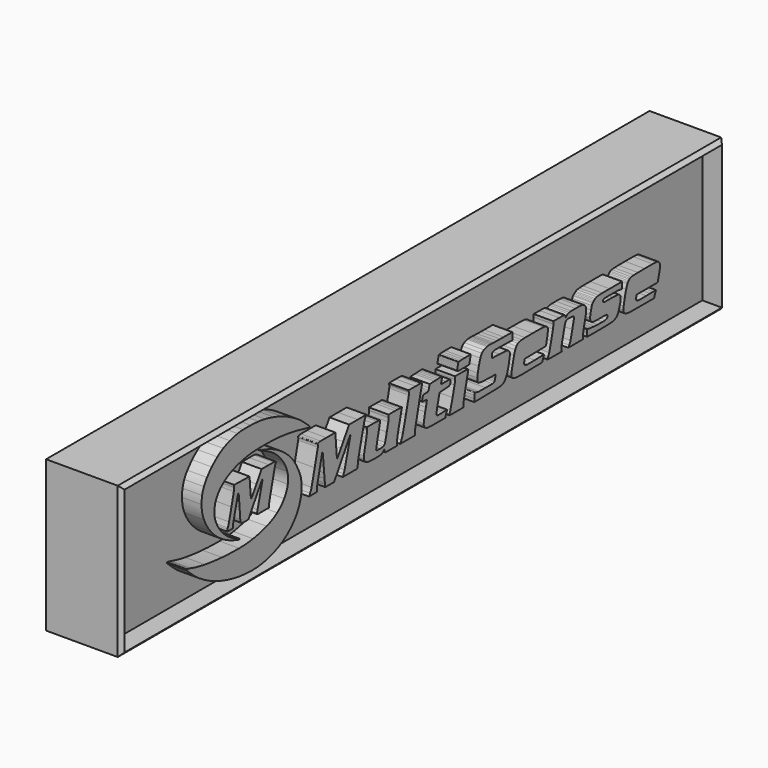
from build123d import *

# Parameters (mm, degrees)
F0_W     = 1000
F0_H     = 200
F1_DEPTH = 100
F2_SIZE  = 5
F3_W     = 990
F3_H     = 190
F4_DEPTH = 26


# Not quite as in the source:
# - ends of sketch curves that miss each other by under 0.0002 mm in the source are joined
# - a feature names something its author has since deleted; it is built from what else it names


with BuildPart() as f1:
    # F0 (on Right) → F1 (new body)
    with BuildSketch(Plane.YZ):
        Rectangle(F0_W, F0_H)
    extrude(amount=F1_DEPTH)

    # F2
    f2_edges = [f1.edges().sort_by_distance(p)[0] for p in [
        (100, 0, 100),
        (100, -500, 0),
        (100, 0, -100),
        (100, 500, 0),
    ]]
    chamfer(f2_edges, length=F2_SIZE)

    # F3 (on face) → F4 (cut)
    with BuildSketch(Plane.YZ.offset(100)):
        Rectangle(F3_W, F3_H)
        with BuildLine():
            ThreePointArc((-246.6238000578, 36.1891009246), (-255.0022324585, 41.7724397208), (-264.0417310007, 46.2063169983))
            ThreePointArc((-264.0417310007, 46.2063169983), (-266.1311900085, 47.0822687591), (-268.2084582005, 47.9867505481))
            ThreePointArc((-268.2084582005, 47.9867505481), (-268.3872731234, 48.2435637092), (-268.2422412968, 48.5208604908))
            ThreePointArc((-268.2422412968, 48.5208604908), (-267.7219027868, 48.7040052158), (-267.1717190083, 48.664106971))
            ThreePointArc((-267.1717190083, 48.664106971), (-264.7541220183, 47.9610524258), (-262.3439659438, 47.2328981825))
            ThreePointArc((-262.3439659438, 47.2328981825), (-255.75593138, 44.9664178565), (-249.3303629782, 42.2736120476))
            ThreePointArc((-249.3303629782, 42.2736120476), (-243.2724946687, 39.2332779494), (-237.4459938241, 35.7701452733))
            ThreePointArc((-237.4459938241, 35.7701452733), (-231.9833169046, 31.9676435498), (-226.8105147999, 27.7793292296))
            ThreePointArc((-226.8105147999, 27.7793292296), (-221.9912407206, 23.2545941628), (-217.5197788497, 18.3858511281))
            ThreePointArc((-217.5197788497, 18.3858511281), (-215.1211615749, 15.3479015259), (-212.9571917947, 12.1385811275))
            ThreePointArc((-212.9571917947, 12.1385811275), (-210.551378863, 8.0777492735), (-208.3170854587, 3.9200787657))
            ThreePointArc((-208.3170854587, 3.9200787657), (-206.3034941374, -0.2333235715), (-204.4645975596, -4.4669698195))
            ThreePointArc((-204.4645975596, -4.4669698195), (-203.2897357301, -7.7656038054), (-202.4281872957, -11.1595720605))
            ThreePointArc((-202.4281872957, -11.1595720605), (-201.4259177378, -22.427417277), (-202.9762712082, -33.6330089467))
            ThreePointArc((-202.9762712082, -33.6330089467), (-207.0222607184, -44.6408161639), (-213.2073987966, -54.6050481569))
            ThreePointArc((-213.2073987966, -54.6050481569), (-221.8366037995, -63.8856917917), (-232.0161676249, -71.4335396171))
            ThreePointArc((-232.0161676249, -71.4335396171), (-244.1370514451, -77.6181065611), (-257.0404061571, -81.9387693814))
            ThreePointArc((-257.0404061571, -81.9387693814), (-270.6114261246, -84.4639864171), (-284.3949819924, -85.2142472745))
            ThreePointArc((-284.3949819924, -85.2142472745), (-299.6324440177, -84.3227142054), (-314.7141769617, -81.9740098137))
            ThreePointArc((-314.7141769617, -81.9740098137), (-330.0151774272, -78.0817139303), (-344.8877120438, -72.782818107))
            ThreePointArc((-344.8877120438, -72.782818107), (-358.728779644, -66.2660528114), (-371.8313622416, -58.368856358))
            ThreePointArc((-371.8313622416, -58.368856358), (-374.9598139965, -56.1511961597), (-377.9827638038, -53.7917467602))
            ThreePointArc((-377.9827638038, -53.7917467602), (-381.6312348274, -50.7314998561), (-385.2042696474, -47.5835046094))
            ThreePointArc((-385.2042696474, -47.5835046094), (-388.7304292554, -44.3731215462), (-392.2297245717, -41.1334775412))
            ThreePointArc((-392.2297245717, -41.1334775412), (-392.4946359393, -40.5378059234), (-392.2503369729, -39.9333880271))
            ThreePointArc((-392.2503369729, -39.9333880271), (-392.0561404098, -39.8152470349), (-391.8293690277, -39.7996141612))
            ThreePointArc((-391.8293690277, -39.7996141612), (-390.9140495548, -39.9639754318), (-390.0013508704, -40.1423163625))
            ThreePointArc((-390.0013508704, -40.1423163625), (-388.9004354267, -40.3814829677), (-387.8062738459, -40.6498594061))
            ThreePointArc((-387.8062738459, -40.6498594061), (-386.5485933112, -40.9877691973), (-385.2969390093, -41.3473590314))
            ThreePointArc((-385.2969390093, -41.3473590314), (-373.7956362594, -44.3337818819), (-362.1164649515, -46.5236776815))
            ThreePointArc((-362.1164649515, -46.5236776815), (-347.8641152603, -48.4083534741), (-333.5490410005, -49.7350500068))
            ThreePointArc((-333.5490410005, -49.7350500068), (-319.2853989301, -50.496519542), (-305.0028930005, -50.6998549053))
            ThreePointArc((-305.0028930005, -50.6998549053), (-293.441650452, -50.2168691086), (-281.9462639341, -48.8933534329))
            ThreePointArc((-281.9462639341, -48.8933534329), (-270.522988434, -46.6581983207), (-259.3285238155, -43.4689815573))
            ThreePointArc((-259.3285238155, -43.4689815573), (-250.3750955195, -39.7652434038), (-242.0511392763, -34.8060796045))
            ThreePointArc((-242.0511392763, -34.8060796045), (-235.7079253752, -29.4741069957), (-230.4110620023, -23.1015459984))
            ThreePointArc((-230.4110620023, -23.1015459984), (-226.6480526025, -16.2091628127), (-224.3981197798, -8.6856670414))
            ThreePointArc((-224.3981197798, -8.6856670414), (-223.9008357191, -1.0084254056), (-225.2628372448, 6.5633829245))
            ThreePointArc((-225.2628372448, 6.5633829245), (-228.5350244194, 14.7357690405), (-233.0907067004, 22.2684222164))
            ThreePointArc((-233.0907067004, 22.2684222164), (-239.3489333395, 29.7229287703), (-246.6238000578, 36.1891009246))
        make_face(mode=Mode.SUBTRACT)
        with BuildLine():
            ThreePointArc((-174.7018401151, 14.0705920271), (-174.5288066312, 15.8520182991), (-174.8362170291, 17.6152309908))
            ThreePointArc((-174.8362170291, 17.6152309908), (-174.8622722087, 18.2073855305), (-174.5871220561, 18.7323790518))
            ThreePointArc((-174.5871220561, 18.7323790518), (-174.0368384738, 19.1539275213), (-173.3770499191, 19.3665164291))
            ThreePointArc((-173.3770499191, 19.3665164291), (-171.798102369, 19.5368741513), (-170.2113269933, 19.6019971351))
            ThreePointArc((-170.2113269933, 19.6019971351), (-165.3776001532, 19.6302348378), (-160.5438, 19.6396489998))
            Line((-160.5438, 19.6396489998), (-145.608858, 19.639649))
            Line((-145.608858, 19.639649), (-144.343966, 3.639649))
            ThreePointArc((-144.343966, 3.639649), (-144.0962884679, 0.5716718243), (-143.8384015545, -2.4954640475))
            ThreePointArc((-143.8384015545, -2.4954640475), (-143.6096761479, -5.0785607207), (-143.36664886, -7.6603510834))
            ThreePointArc((-143.36664886, -7.6603510834), (-143.1436912653, -9.9532312874), (-142.919313494, -12.2459729503))
            ThreePointArc((-142.919313494, -12.2459729503), (-142.8783010175, -12.327499768), (-142.793157, -12.360351))
            ThreePointArc((-142.793157, -12.360351), (-142.6920587596, -12.3343745217), (-142.6160043003, -12.2628808097))
            ThreePointArc((-142.6160043003, -12.2628808097), (-141.1591567944, -9.9628213076), (-139.7031838583, -7.6622080896))
            ThreePointArc((-139.7031838583, -7.6622080896), (-138.0793333583, -5.0838383234), (-136.4658248264, -2.4989841079))
            ThreePointArc((-136.4658248264, -2.4989841079), (-134.5669888164, 0.5648690609), (-132.6756031958, 3.6333271203))
            Line((-132.6756031958, 3.6333271203), (-122.843966, 19.627006))
            Line((-122.843966, 19.627006), (-108.570914, 19.633327))
            Line((-108.570914, 19.633327), (-94.297861, 19.639649))
            Line((-94.297861, 19.639649), (-95.759344, 17.389649))
            ThreePointArc((-95.759344, 17.389649), (-96.8435272527, 15.3828466119), (-97.5910089736, 13.2278569932))
            ThreePointArc((-97.5910089736, 13.2278569932), (-100.2300256588, 2.944764842), (-102.8292478626, -7.3484580344))
            ThreePointArc((-102.8292478626, -7.3484580344), (-105.3240499629, -17.4199326533), (-107.7666081157, -27.5042049723))
            ThreePointArc((-107.7666081157, -27.5042049723), (-108.3156162068, -30.5257876099), (-108.5276931669, -33.5895099977))
            Line((-108.5276931669, -33.5895099977), (-108.579734, -37.360351))
            Line((-108.579734, -37.360351), (-120.945672, -37.360351))
            Line((-120.945672, -37.360351), (-133.311609, -37.360351))
            Line((-133.311609, -37.360351), (-131.786789, -34.110351))
            ThreePointArc((-131.786789, -34.110351), (-130.9369585949, -32.0751860313), (-130.2655961338, -29.9743812362))
            ThreePointArc((-130.2655961338, -29.9743812362), (-127.9075333412, -21.2798219374), (-125.5730053742, -12.5789139002))
            ThreePointArc((-125.5730053742, -12.5789139002), (-123.0704426319, -3.1909836778), (-120.5728943872, 6.1982818372))
            ThreePointArc((-120.5728943872, 6.1982818372), (-120.6339116845, 6.5025434885), (-120.9123, 6.639649))
            ThreePointArc((-120.9123, 6.639649), (-121.0170732669, 6.6123791239), (-121.0952571029, 6.5374900634))
            ThreePointArc((-121.0952571029, 6.5374900634), (-123.05447176, 3.3575349389), (-125.0129869412, 0.1771489638))
            ThreePointArc((-125.0129869412, 0.1771489638), (-127.1897075437, -3.3705687245), (-129.3555760622, -6.9249219623))
            ThreePointArc((-129.3555760622, -6.9249219623), (-131.9100848721, -11.1402796116), (-134.4567992039, -15.3603508772))
            Line((-134.4567992039, -15.3603508772), (-147.705562, -37.360351))
            Line((-147.705562, -37.360351), (-154.979451, -37.360351))
            Line((-154.979451, -37.360351), (-162.25334, -37.360351))
            Line((-162.25334, -37.360351), (-162.760776, -34.110351))
            ThreePointArc((-162.760776, -34.110351), (-162.9107585781, -33.0591277623), (-163.0330110102, -32.004320001))
            ThreePointArc((-163.0330110102, -32.004320001), (-163.3101001353, -29.273344058), (-163.5811588046, -26.5417629808))
            ThreePointArc((-163.5811588046, -26.5417629808), (-163.8961688648, -23.2819197125), (-164.2015999848, -20.0211649986))
            ThreePointArc((-164.2015999848, -20.0211649986), (-164.5253336731, -16.465332125), (-164.8410009488, -12.9087740831))
            ThreePointArc((-164.8410009488, -12.9087740831), (-165.1490364856, -9.4551931792), (-165.4679088818, -6.0025959889))
            ThreePointArc((-165.4679088818, -6.0025959889), (-165.7511968306, -3.0669928077), (-166.0493879522, -0.132865995))
            ThreePointArc((-166.0493879522, -0.132865995), (-166.3208571519, 2.4624010871), (-166.5944230956, 5.0574479899))
            ThreePointArc((-166.5944230956, 5.0574479899), (-166.6429829681, 5.2292792572), (-166.7460646389, 5.3750813611))
            ThreePointArc((-166.7460646389, 5.3750813611), (-167.0844597869, 5.4636849239), (-167.3275310693, 5.2121330169))
            ThreePointArc((-167.3275310693, 5.2121330169), (-169.5531744189, -3.9427367497), (-171.7704491797, -13.0996369566))
            ThreePointArc((-171.7704491797, -13.0996369566), (-173.838625297, -21.7166592084), (-175.8799409879, -30.3400840029))
            ThreePointArc((-175.8799409879, -30.3400840029), (-176.2275732978, -32.3275396649), (-176.343966, -34.341809))
            Line((-176.343966, -34.341809), (-176.343966, -37.360351))
            Line((-176.343966, -37.360351), (-182.810241, -37.360351))
            Line((-182.810241, -37.360351), (-189.276516, -37.360351))
            Line((-189.276516, -37.360351), (-187.423727, -34.110351))
            ThreePointArc((-187.423727, -34.110351), (-186.0478869675, -31.2722635114), (-185.0619934039, -28.2763178964))
            ThreePointArc((-185.0619934039, -28.2763178964), (-182.4403880481, -17.925494631), (-179.8833388541, -7.5585347922))
            ThreePointArc((-179.8833388541, -7.5585347922), (-177.2732199659, 3.2513884324), (-174.7018401151, 14.0705920271))
        make_face(mode=Mode.SUBTRACT)
        with BuildLine():
            ThreePointArc((-92.8820085608, 0.7789769433), (-92.8555492874, 1.5381745527), (-92.9708167067, 2.2890370736))
            Line((-92.9708167067, 2.2890370736), (-93.560783, 4.639649))
            Line((-93.560783, 4.639649), (-82.452375, 4.639649))
            ThreePointArc((-82.452375, 4.639649), (-79.5692857083, 4.6256589691), (-76.6864680002, 4.5836869916))
            ThreePointArc((-76.6864680002, 4.5836869916), (-75.1287207374, 4.5121189787), (-73.5769520517, 4.3581305901))
            ThreePointArc((-73.5769520517, 4.3581305901), (-72.7019959607, 4.2003743806), (-71.8486289714, 3.9509750816))
            ThreePointArc((-71.8486289714, 3.9509750816), (-71.4829329227, 3.675455544), (-71.343966, 3.239184))
            ThreePointArc((-71.343966, 3.239184), (-71.370292438, 2.7365856799), (-71.4489819583, 2.2394879911))
            ThreePointArc((-71.4489819583, 2.2394879911), (-71.9091414316, 0.0885075025), (-72.3754332875, -2.0611519372))
            ThreePointArc((-72.3754332875, -2.0611519372), (-72.9352375059, -4.5885887792), (-73.5098987944, -7.1126890475))
            ThreePointArc((-73.5098987944, -7.1126890475), (-74.1768670893, -9.9766475695), (-74.8553424273, -12.8379018978))
            ThreePointArc((-74.8553424273, -12.8379018978), (-75.5211841502, -15.6807219843), (-76.1599101484, -18.5297569675))
            ThreePointArc((-76.1599101484, -18.5297569675), (-76.6819973595, -20.9983559149), (-77.1676976513, -23.4743710657))
            ThreePointArc((-77.1676976513, -23.4743710657), (-77.5591822036, -25.5855429243), (-77.9380302439, -27.699018957))
            ThreePointArc((-77.9380302439, -27.699018957), (-77.9351205503, -28.0812660319), (-77.7963248707, -28.4374359201))
            ThreePointArc((-77.7963248707, -28.4374359201), (-77.1639553329, -29.0550222177), (-76.316013967, -29.3046202272))
            ThreePointArc((-76.316013967, -29.3046202272), (-73.8072006791, -29.3687719786), (-71.2976590017, -29.3473199346))
            ThreePointArc((-71.2976590017, -29.3473199346), (-68.7967844857, -29.2369885562), (-66.3016960138, -29.034306862))
            ThreePointArc((-66.3016960138, -29.034306862), (-65.3291404192, -28.7396605794), (-64.5411655861, -28.0979623435))
            ThreePointArc((-64.5411655861, -28.0979623435), (-63.7291730222, -26.8688900483), (-63.2019316871, -25.4934020823))
            ThreePointArc((-63.2019316871, -25.4934020823), (-61.7711663359, -19.9665618492), (-60.3827667736, -14.4289270559))
            ThreePointArc((-60.3827667736, -14.4289270559), (-59.0917996717, -9.058422133), (-57.8645512293, -3.6729991708))
            ThreePointArc((-57.8645512293, -3.6729991708), (-57.4745015081, -1.3101306124), (-57.343966, 1.081155))
            Line((-57.343966, 1.081155), (-57.343966, 4.639649))
            Line((-57.343966, 4.639649), (-46.343966, 4.639649))
            ThreePointArc((-46.343966, 4.639649), (-44.2349572127, 4.6315456778), (-42.1260730001, 4.607232993))
            ThreePointArc((-42.1260730001, 4.607232993), (-40.3503241981, 4.568564733), (-38.5752160227, 4.5071644458))
            ThreePointArc((-38.5752160227, 4.5071644458), (-37.0467998485, 4.4419856165), (-35.5186059933, 4.3717871409))
            ThreePointArc((-35.5186059933, 4.3717871409), (-35.3946240422, 4.3151724942), (-35.343966, 4.18864))
            ThreePointArc((-35.343966, 4.18864), (-35.3545141697, 4.0101720375), (-35.3860111042, 3.8341890251))
            ThreePointArc((-35.3860111042, 3.8341890251), (-36.0240723623, 1.1839431843), (-36.6628125832, -1.4661391005))
            ThreePointArc((-36.6628125832, -1.4661391005), (-37.3850371054, -4.4495014263), (-38.1124575639, -7.4316011068))
            ThreePointArc((-38.1124575639, -7.4316011068), (-38.9711650013, -10.9304366782), (-39.8336576195, -14.428341094))
            ThreePointArc((-39.8336576195, -14.428341094), (-40.7224324489, -18.1079758675), (-41.5722052918, -21.7968129344))
            ThreePointArc((-41.5722052918, -21.7968129344), (-42.2538172532, -24.9539682129), (-42.8817329773, -28.1222400043))
            ThreePointArc((-42.8817329773, -28.1222400043), (-43.3537772844, -30.6981676106), (-43.7952699566, -33.2795070072))
            ThreePointArc((-43.7952699566, -33.2795070072), (-43.8474447965, -34.132015094), (-43.7252498407, -34.97733196))
            Line((-43.7252498407, -34.97733196), (-43.12715, -37.360351))
            Line((-43.12715, -37.360351), (-53.735558, -37.360351))
            ThreePointArc((-53.735558, -37.360351), (-57.0528891948, -37.3489981413), (-60.370065, -37.3149419997))
            ThreePointArc((-60.370065, -37.3149419997), (-61.5978913503, -37.2430294131), (-62.8143529612, -37.0615078014))
            ThreePointArc((-62.8143529612, -37.0615078014), (-63.4156948753, -36.8372007938), (-63.9126482503, -36.4310442202))
            ThreePointArc((-63.9126482503, -36.4310442202), (-64.2325506019, -35.8987350586), (-64.343966, -35.287771))
            Line((-64.343966, -35.287771), (-64.343966, -33.215191))
            Line((-64.343966, -33.215191), (-66.978825, -35.287771))
            ThreePointArc((-66.978825, -35.287771), (-67.8685341553, -35.8968315763), (-68.8308879846, -36.3830540362))
            ThreePointArc((-68.8308879846, -36.3830540362), (-69.8772441586, -36.7542771754), (-70.9608460238, -36.9960928517))
            ThreePointArc((-70.9608460238, -36.9960928517), (-72.5340330575, -37.1945000905), (-74.1169599875, -37.2873724962))
            ThreePointArc((-74.1169599875, -37.2873724962), (-77.0151132985, -37.3421068265), (-79.913726, -37.360351))
            ThreePointArc((-79.913726, -37.360351), (-86.0337872387, -37.1577677784), (-92.1270539965, -36.5508989738))
            ThreePointArc((-92.1270539965, -36.5508989738), (-94.9544039084, -35.5060432796), (-97.0603997841, -33.3495618671))
            ThreePointArc((-97.0603997841, -33.3495618671), (-98.2670877075, -30.2774313015), (-98.3296614975, -26.9774060804))
            ThreePointArc((-98.3296614975, -26.9774060804), (-96.9946010963, -19.5944839615), (-95.3624083293, -12.2715151638))
            ThreePointArc((-95.3624083293, -12.2715151638), (-94.7928779635, -9.8521718155), (-94.2636129331, -7.423702014))
            ThreePointArc((-94.2636129331, -7.423702014), (-93.8225243645, -5.1952582662), (-93.4299855296, -2.9577520773))
            ThreePointArc((-93.4299855296, -2.9577520773), (-93.1399396448, -1.091742323), (-92.8820085608, 0.7789769433))
        make_face(mode=Mode.SUBTRACT)
        with BuildLine():
            ThreePointArc((-23.7762746869, 13.4799029263), (-23.5592137009, 15.4111581767), (-23.8046477922, 17.3390130522))
            Line((-23.8046477922, 17.3390130522), (-24.382071, 19.639649))
            Line((-24.382071, 19.639649), (-12.795631, 19.639649))
            ThreePointArc((-12.795631, 19.639649), (-9.3252799803, 19.6286241096), (-5.855069, 19.5955559945))
            ThreePointArc((-5.855069, 19.5955559945), (-4.4845108182, 19.5286755978), (-3.1223320904, 19.3632314288))
            ThreePointArc((-3.1223320904, 19.3632314288), (-2.5163729631, 19.1737950727), (-1.99065478, 18.8178552404))
            ThreePointArc((-1.99065478, 18.8178552404), (-1.7291495383, 18.3905713906), (-1.7349010858, 17.8896490258))
            ThreePointArc((-1.7349010858, 17.8896490258), (-3.3928563764, 12.0967018693), (-4.8987388064, 6.2623749527))
            ThreePointArc((-4.8987388064, 6.2623749527), (-7.1399664187, -3.0567092726), (-9.3159254042, -12.3912491367))
            ThreePointArc((-9.3159254042, -12.3912491367), (-11.6228722462, -22.4865787129), (-13.9124309628, -32.5858660084))
            ThreePointArc((-13.9124309628, -32.5858660084), (-14.0431451519, -33.8252115665), (-13.882940485, -35.0610911217))
            Line((-13.882940485, -35.0610911217), (-13.305862, -37.360351))
            Line((-13.305862, -37.360351), (-25.741836, -37.360351))
            Line((-25.741836, -37.360351), (-38.177809, -37.360351))
            Line((-38.177809, -37.360351), (-36.238293, -33.610351))
            ThreePointArc((-36.238293, -33.610351), (-34.8029111414, -30.4085359201), (-33.7335388308, -27.0666227845))
            ThreePointArc((-33.7335388308, -27.0666227845), (-31.2057732248, -17.1754751895), (-28.7495673815, -7.2663151509))
            ThreePointArc((-28.7495673815, -7.2663151509), (-26.2417602548, 3.1017212165), (-23.7762746869, 13.4799029263))
        make_face(mode=Mode.SUBTRACT)
        with BuildLine():
            Line((10.710733, 12.556505), (18.433383, 12.896833))
            ThreePointArc((18.433383, 12.896833), (20.0150642394, 12.9679512677), (21.596615969, 13.0418936503))
            ThreePointArc((21.596615969, 13.0418936503), (23.1559363779, 13.1176473578), (24.715112999, 13.1963050186))
            ThreePointArc((24.715112999, 13.1963050186), (26.0626915551, 13.2667548968), (27.4101419959, 13.3396140744))
            ThreePointArc((27.4101419959, 13.3396140744), (28.1919839798, 13.3858054393), (28.9734210088, 13.4384048769))
            ThreePointArc((28.9734210088, 13.4384048769), (29.6976088145, 13.4731927642), (30.4226309997, 13.4741979855))
            ThreePointArc((30.4226309997, 13.4741979855), (30.7902926142, 13.4130817803), (31.1258412809, 13.2508554167))
            ThreePointArc((31.1258412809, 13.2508554167), (31.3197344674, 13.0368328391), (31.3920117775, 12.7572329975))
            ThreePointArc((31.3920117775, 12.7572329975), (31.364075691, 12.3188883561), (31.2709087364, 11.8896490783))
            ThreePointArc((31.2709087364, 11.8896490783), (31.1458342195, 11.459339518), (31.0258569283, 11.0275810195))
            ThreePointArc((31.0258569283, 11.0275810195), (30.8670476848, 10.4371158375), (30.7110607049, 9.8458988158))
            ThreePointArc((30.7110607049, 9.8458988158), (30.546168436, 9.2086756782), (30.3842906061, 8.5706800989))
            ThreePointArc((30.3842906061, 8.5706800989), (30.2379327035, 7.9805977161), (30.0951134781, 7.389648886))
            Line((30.0951134781, 7.389648886), (29.439217, 4.639649))
            Line((29.439217, 4.639649), (37.547625, 4.639649))
            ThreePointArc((37.547625, 4.639649), (40.3846536738, 4.6181373748), (43.2210299998, 4.5536099928))
            ThreePointArc((43.2210299998, 4.5536099928), (44.091879106, 4.4003477995), (44.8834241203, 4.0062361737))
            ThreePointArc((44.8834241203, 4.0062361737), (45.3274898932, 3.4660091937), (45.4210098662, 2.7729768755))
            ThreePointArc((45.4210098662, 2.7729768755), (45.1428706372, 1.1958949639), (44.7651836678, -0.3603509081))
            ThreePointArc((44.7651836678, -0.3603509081), (44.4787720848, -1.1055569362), (44.053955451, -1.7814965755))
            ThreePointArc((44.053955451, -1.7814965755), (43.5557336364, -2.2585180802), (42.9394438694, -2.5682946015))
            ThreePointArc((42.9394438694, -2.5682946015), (41.9011377378, -2.8422885504), (40.8378520611, -2.992541747))
            ThreePointArc((40.8378520611, -2.992541747), (38.2273937691, -3.1911541636), (35.6148640133, -3.3603512243))
            Line((35.6148640133, -3.3603512243), (27.156034, -3.860351))
            Line((27.156034, -3.860351), (24.280417, -15.061808))
            ThreePointArc((24.280417, -15.061808), (23.7346435132, -17.2637643568), (23.2256231964, -19.4745060435))
            ThreePointArc((23.2256231964, -19.4745060435), (22.8088263115, -21.4648580691), (22.4381073986, -23.4643050692))
            ThreePointArc((22.4381073986, -23.4643050692), (22.1636104377, -25.1274252753), (21.9164414026, -26.7948259164))
            ThreePointArc((21.9164414026, -26.7948259164), (21.9091352355, -27.3738679131), (22.0468226355, -27.9363491399))
            ThreePointArc((22.0468226355, -27.9363491399), (22.3386717688, -28.4253348004), (22.778110796, -28.7875173583))
            ThreePointArc((22.778110796, -28.7875173583), (23.4130165524, -29.0723124155), (24.0905920074, -29.2307579453))
            ThreePointArc((24.0905920074, -29.2307579453), (25.2636051995, -29.3404719811), (26.4416490008, -29.3549610301))
            ThreePointArc((26.4416490008, -29.3549610301), (28.8076224929, -29.2739021398), (31.1724389675, -29.1641563807))
            ThreePointArc((31.1724389675, -29.1641563807), (32.7987235905, -29.084196737), (34.4255020073, -29.0150071859))
            ThreePointArc((34.4255020073, -29.0150071859), (35.7945268348, -28.9689041736), (37.1639780028, -28.9379531627))
            ThreePointArc((37.1639780028, -28.9379531627), (38.3512231605, -28.9191532629), (39.5385110035, -28.9032762879))
            ThreePointArc((39.5385110035, -28.9032762879), (39.6215252549, -28.9367787024), (39.656034, -29.01938))
            ThreePointArc((39.656034, -29.01938), (39.6463338481, -29.1297105738), (39.6175310109, -29.236656004))
            ThreePointArc((39.6175310109, -29.236656004), (39.401349129, -29.8249087899), (39.1835134741, -30.4125511765))
            ThreePointArc((39.1835134741, -30.4125511765), (38.9262061123, -31.0960536051), (38.6639196535, -31.7776608652))
            ThreePointArc((38.6639196535, -31.7776608652), (38.3575660447, -32.5596293768), (38.0474541934, -33.3401150774))
            Line((38.0474541934, -33.3401150774), (36.438874, -37.360351))
            Line((36.438874, -37.360351), (21.797454, -37.345609))
            ThreePointArc((21.797454, -37.345609), (14.5856128269, -37.21489465), (7.3824699999, -36.8374390019))
            ThreePointArc((7.3824699999, -36.8374390019), (4.6306871326, -36.1014529812), (2.3545863418, -34.3887506918))
            ThreePointArc((2.3545863418, -34.3887506918), (1.028190726, -32.0348751477), (0.8345160223, -29.3399640034))
            ThreePointArc((0.8345160223, -29.3399640034), (1.9263065335, -23.0638613747), (3.3090337449, -16.845377937))
            ThreePointArc((3.3090337449, -16.845377937), (3.8894632412, -14.44664571), (4.4474681486, -12.0425980338))
            ThreePointArc((4.4474681486, -12.0425980338), (4.8998730149, -9.9805327187), (5.3215791103, -7.9119710216))
            ThreePointArc((5.3215791103, -7.9119710216), (5.6645530824, -6.1393451569), (5.9984605398, -4.3649891002))
            ThreePointArc((5.9984605398, -4.3649891002), (5.983357001, -4.1082460813), (5.8504259012, -3.8880770988))
            ThreePointArc((5.8504259012, -3.8880770988), (5.6673300333, -3.7538209138), (5.4523398841, -3.6808276571))
            ThreePointArc((5.4523398841, -3.6808276571), (4.8932697474, -3.5902554251), (4.3318829117, -3.5153717412))
            ThreePointArc((4.3318829117, -3.5153717412), (3.6441989404, -3.4453250825), (2.9545219902, -3.3988331944))
            ThreePointArc((2.9545219902, -3.3988331944), (2.1884920325, -3.3699729877), (1.421979, -3.360351))
            ThreePointArc((1.421979, -3.360351), (0.261336254, -3.3458210387), (-0.8985790006, -3.3022400119))
            ThreePointArc((-0.8985790006, -3.3022400119), (-1.352755268, -3.2154594429), (-1.7657931394, -3.0075972015))
            ThreePointArc((-1.7657931394, -3.0075972015), (-1.9963892518, -2.736789198), (-2.0616291222, -2.3871389907))
            ThreePointArc((-2.0616291222, -2.3871389907), (-1.9793888036, -1.7428873532), (-1.8320069445, -1.110351016))
            ThreePointArc((-1.8320069445, -1.110351016), (-1.6901315737, -0.6158196359), (-1.5487593322, -0.1211441905))
            ThreePointArc((-1.5487593322, -0.1211441905), (-1.3901255446, 0.4357584041), (-1.2318888791, 0.9927739657))
            ThreePointArc((-1.2318888791, 0.9927739657), (-1.0807996236, 1.5260852151), (-0.9300941355, 2.0595050382))
            ThreePointArc((-0.9300941355, 2.0595050382), (-0.8133499366, 2.4744891832), (-0.6972323157, 2.889649088))
            ThreePointArc((-0.6972323157, 2.889649088), (-0.5089931607, 3.3363654033), (-0.2146736319, 3.7215476363))
            ThreePointArc((-0.2146736319, 3.7215476363), (0.1788107925, 4.0395286756), (0.6330221023, 4.2623157147))
            ThreePointArc((0.6330221023, 4.2623157147), (1.310086198, 4.4550723302), (2.0067980417, 4.5558864592))
            ThreePointArc((2.0067980417, 4.5558864592), (3.0950325043, 4.6187004453), (4.184877, 4.639649))
            ThreePointArc((4.184877, 4.639649), (5.5593457023, 4.6645053623), (6.9320169997, 4.7390410044))
            ThreePointArc((6.9320169997, 4.7390410044), (7.5606856151, 4.8737419202), (8.1284056928, 5.1755074237))
            ThreePointArc((8.1284056928, 5.1755074237), (8.5755766224, 5.6141161483), (8.8748869919, 6.1643460029))
            ThreePointArc((8.8748869919, 6.1643460029), (9.2862561727, 7.372861573), (9.6448395828, 8.5980768431))
            Line((9.6448395828, 8.5980768431), (10.710733, 12.556505))
        make_face(mode=Mode.SUBTRACT)
        with BuildLine():
            ThreePointArc((51.9022226579, -5.2582841539), (52.4389392331, -2.2047165976), (52.6319187135, 0.8896489954))
            Line((52.6319187135, 0.8896489954), (52.656034, 4.639649))
            Line((52.656034, 4.639649), (63.656034, 4.639649))
            ThreePointArc((63.656034, 4.639649), (65.7713867516, 4.6230743653), (67.8862199998, 4.5733519931))
            ThreePointArc((67.8862199998, 4.5733519931), (69.6616689356, 4.4943099293), (71.4344260008, 4.3686160101))
            ThreePointArc((71.4344260008, 4.3686160101), (72.8798924917, 4.2371149993), (74.3234390522, 4.0859884682))
            ThreePointArc((74.3234390522, 4.0859884682), (74.5607496726, 3.9636371385), (74.656034, 3.714224))
            ThreePointArc((74.656034, 3.714224), (74.6364681199, 3.3636478568), (74.5780139398, 3.0174260137))
            ThreePointArc((74.5780139398, 3.0174260137), (74.0309050223, 0.6113211442), (73.481034099, -1.7941540227))
            ThreePointArc((73.481034099, -1.7941540227), (72.8401879658, -4.5667356489), (72.1891210211, -7.336935005))
            ThreePointArc((72.1891210211, -7.336935005), (71.4264049284, -10.5384676643), (70.6560334922, -13.7381668771))
            ThreePointArc((70.6560334922, -13.7381668771), (69.8752918773, -17.0288402619), (69.1242686935, -20.3264231547))
            ThreePointArc((69.1242686935, -20.3264231547), (68.4602382736, -23.3857590873), (67.8310344937, -26.4524470984))
            ThreePointArc((67.8310344937, -26.4524470984), (67.3304609253, -29.0261230424), (66.853498345, -31.6042790622))
            ThreePointArc((66.853498345, -31.6042790622), (66.7054984882, -32.7041053724), (66.656034, -33.812742))
            Line((66.656034, -33.812742), (66.656034, -37.360351))
            Line((66.656034, -37.360351), (54.001046, -37.360351))
            ThreePointArc((54.001046, -37.360351), (49.8256140078, -37.3524363883), (45.650242, -37.3286970033))
            ThreePointArc((45.650242, -37.3286970033), (44.437536723, -37.268497216), (43.2341640634, -37.1067186427))
            ThreePointArc((43.2341640634, -37.1067186427), (42.8498789018, -36.8847953207), (42.6973037951, -36.4680869977))
            ThreePointArc((42.6973037951, -36.4680869977), (42.7999718044, -35.9092440698), (43.0974155878, -35.4251226269))
            ThreePointArc((43.0974155878, -35.4251226269), (44.189990847, -33.8953482119), (44.9037659099, -32.1562519747))
            ThreePointArc((44.9037659099, -32.1562519747), (46.7854797427, -25.3508201594), (48.608120887, -18.5293299703))
            ThreePointArc((48.608120887, -18.5293299703), (50.2998154125, -11.904888384), (51.9022226579, -5.2582841539))
        make_face(mode=Mode.SUBTRACT)
        with BuildLine():
            ThreePointArc((100.5295100738, 16.0131548456), (103.0415445388, 17.0386409142), (105.65603404, 17.7641638142))
            ThreePointArc((105.65603404, 17.7641638142), (106.4991246537, 17.9195002611), (107.350021053, 18.023934426))
            ThreePointArc((107.350021053, 18.023934426), (108.4723511936, 18.1123019785), (109.5966590022, 18.1703169422))
            ThreePointArc((109.5966590022, 18.1703169422), (110.7909264953, 18.1998534661), (111.9855570093, 18.1975716083))
            ThreePointArc((111.9855570093, 18.1975716083), (113.0717664629, 18.1618200327), (114.1560340366, 18.0877054252))
            ThreePointArc((114.1560340366, 18.0877054252), (115.5548441002, 17.9855918344), (116.9558429763, 17.9200252975))
            ThreePointArc((116.9558429763, 17.9200252975), (119.4143427098, 17.8438132502), (121.873221006, 17.7809902629))
            ThreePointArc((121.873221006, 17.7809902629), (124.7283479867, 17.7239846599), (127.5837540034, 17.6832882992))
            ThreePointArc((127.5837540034, 17.6832882992), (130.4948468946, 17.6579665945), (133.4060340003, 17.6483415264))
            Line((133.4060340003, 17.6483415264), (147.656034, 17.639649))
            Line((147.656034, 17.639649), (147.65739, 12.889649))
            Line((147.65739, 12.889649), (147.658747, 8.139649))
            Line((147.658747, 8.139649), (131.510187, 8.460487))
            ThreePointArc((131.510187, 8.460487), (125.7446533288, 8.5496104654), (119.9785580017, 8.5879017535))
            ThreePointArc((119.9785580017, 8.5879017535), (118.0060996882, 8.457012912), (116.069991987, 8.0580010467))
            ThreePointArc((116.069991987, 8.0580010467), (115.0223407929, 7.4945976298), (114.3176576957, 6.5362561331))
            ThreePointArc((114.3176576957, 6.5362561331), (113.8391511172, 5.0461254607), (113.6713458108, 3.4900730011))
            Line((113.6713458108, 3.4900730011), (113.656034, 0.840496))
            Line((113.656034, 0.840496), (126.552107, 0.490073))
            ThreePointArc((126.552107, 0.490073), (132.4166879534, 0.2185749712), (138.2666260544, -0.2766474761))
            ThreePointArc((138.2666260544, -0.2766474761), (140.5775855275, -0.9869885598), (142.4459771491, -2.5213388773))
            ThreePointArc((142.4459771491, -2.5213388773), (143.5383394027, -4.6135309115), (143.6948703055, -6.9685300434))
            ThreePointArc((143.6948703055, -6.9685300434), (142.7951223654, -12.437912328), (141.6555565253, -17.8624011225))
            ThreePointArc((141.6555565253, -17.8624011225), (140.7863479307, -21.3236081342), (139.800228599, -24.7533378773))
            ThreePointArc((139.800228599, -24.7533378773), (138.9077167203, -27.3200355215), (137.8243096525, -29.8121718331))
            ThreePointArc((137.8243096525, -29.8121718331), (136.8010845241, -31.69386579), (135.5942133144, -33.4633922384))
            ThreePointArc((135.5942133144, -33.4633922384), (134.3809048548, -34.8180485171), (132.963638626, -35.9575954481))
            ThreePointArc((132.963638626, -35.9575954481), (131.7971695222, -36.60086362), (130.5329949351, -37.0207527217))
            ThreePointArc((130.5329949351, -37.0207527217), (128.7215510963, -37.3755978395), (126.8894559524, -37.6007004524))
            ThreePointArc((126.8894559524, -37.6007004524), (123.8017236513, -37.818881358), (120.7085640029, -37.9374441291))
            ThreePointArc((120.7085640029, -37.9374441291), (114.0575466008, -38.0713915032), (107.4060340007, -38.1779490495))
            Line((107.4060340007, -38.1779490495), (84.656034, -38.495547))
            Line((84.656034, -38.495547), (84.656034, -34.509737))
            ThreePointArc((84.656034, -34.509737), (84.6906957788, -32.5638684269), (84.7946409775, -30.6204689984))
            ThreePointArc((84.7946409775, -30.6204689984), (84.9767790337, -29.665087423), (85.3757192235, -28.7780841339))
            ThreePointArc((85.3757192235, -28.7780841339), (85.8497016226, -28.3068419901), (86.4910260052, -28.1186091411))
            ThreePointArc((86.4910260052, -28.1186091411), (87.4136223819, -28.1768968912), (88.3062119406, -28.4174491563))
            ThreePointArc((88.3062119406, -28.4174491563), (90.1680213505, -28.9504395647), (92.0929549996, -29.1626740139))
            ThreePointArc((92.0929549996, -29.1626740139), (97.715339469, -29.2740774752), (103.3386089994, -29.3236521689))
            ThreePointArc((103.3386089994, -29.3236521689), (109.1158139906, -29.3202054924), (114.8928149989, -29.2715359084))
            ThreePointArc((114.8928149989, -29.2715359084), (116.2198381959, -29.0701558626), (117.4414650641, -28.5141231011))
            ThreePointArc((117.4414650641, -28.5141231011), (117.7410347983, -28.2704332081), (117.9756306513, -27.9636897931))
            ThreePointArc((117.9756306513, -27.9636897931), (118.2654069182, -27.4358777798), (118.5193949174, -26.8899419649))
            ThreePointArc((118.5193949174, -26.8899419649), (118.7756062656, -26.2304178458), (118.9896534742, -25.5560291342))
            ThreePointArc((118.9896534742, -25.5560291342), (119.1682719483, -24.8477120457), (119.3059382678, -24.1303100435))
            Line((119.3059382678, -24.1303100435), (119.884979, -20.562099))
            Line((119.884979, -20.562099), (106.422645, -20.211225))
            ThreePointArc((106.422645, -20.211225), (103.265289717, -20.1110871227), (100.109266993, -19.9752911442))
            ThreePointArc((100.109266993, -19.9752911442), (97.9208404578, -19.8331313113), (95.738175993, -19.6200680618))
            ThreePointArc((95.738175993, -19.6200680618), (94.2180564121, -19.4160786325), (92.7072410466, -19.1518587614))
            ThreePointArc((92.7072410466, -19.1518587614), (91.9659761488, -18.9078159368), (91.3081717138, -18.4879063445))
            ThreePointArc((91.3081717138, -18.4879063445), (90.4642554585, -17.4931341544), (90.0103403548, -16.270134935))
            ThreePointArc((90.0103403548, -16.270134935), (89.7684464348, -14.3444739135), (89.744678692, -12.4038249864))
            ThreePointArc((89.744678692, -12.4038249864), (89.9727203949, -9.6655768271), (90.4133166368, -6.9534041291))
            ThreePointArc((90.4133166368, -6.9534041291), (91.2208229269, -3.2637113827), (92.1418261099, 0.3992999706))
            ThreePointArc((92.1418261099, 0.3992999706), (93.3571489686, 4.6193595203), (94.7288969483, 8.7911960181))
            ThreePointArc((94.7288969483, 8.7911960181), (95.7822046145, 11.1653271465), (97.2057610473, 13.3377549632))
            ThreePointArc((97.2057610473, 13.3377549632), (98.7119556124, 14.8688619001), (100.5295100738, 16.0131548456))
        make_face(mode=Mode.SUBTRACT)
        with BuildLine():
            ThreePointArc((154.5197259763, -1.5655859823), (155.678247307, -0.2902674462), (157.0573020505, 0.7426009172))
            ThreePointArc((157.0573020505, 0.7426009172), (158.2839344004, 1.3626859083), (159.5933010597, 1.7806467443))
            ThreePointArc((159.5933010597, 1.7806467443), (161.3324419768, 2.1181259285), (163.0920979874, 2.3233431606))
            ThreePointArc((163.0920979874, 2.3233431606), (165.9897201618, 2.5005021014), (168.8917290038, 2.5776005966))
            ThreePointArc((168.8917290038, 2.5776005966), (175.0375614404, 2.6207868168), (181.183527, 2.6359107274))
            ThreePointArc((181.183527, 2.6359107274), (190.3391485401, 2.5652329089), (199.4925119963, 2.3499688817))
            ThreePointArc((199.4925119963, 2.3499688817), (202.3426122614, 1.841193963), (204.9275899249, 0.537424893))
            ThreePointArc((204.9275899249, 0.537424893), (206.4160111998, -1.2591588804), (206.7848096004, -3.5628729567))
            ThreePointArc((206.7848096004, -3.5628729567), (206.0485092869, -8.8527807531), (204.9912761826, -14.0880000427))
            Line((204.9912761826, -14.0880000427), (203.300885, -21.315648))
            Line((203.300885, -21.315648), (185.799529, -21.588))
            Line((185.799529, -21.588), (168.298172, -21.860351))
            Line((168.298172, -21.860351), (167.512668, -24.800741))
            ThreePointArc((167.512668, -24.800741), (167.2926173099, -26.3691537763), (167.4569057523, -27.9443840568))
            ThreePointArc((167.4569057523, -27.9443840568), (168.0201442261, -29.0109428313), (169.0392591669, -29.656070468))
            ThreePointArc((169.0392591669, -29.656070468), (171.1192751148, -30.1399230437), (173.2484090009, -30.3053575634))
            ThreePointArc((173.2484090009, -30.3053575634), (178.9757738302, -30.2835462988), (184.702492006, -30.1947622826))
            Line((184.702492006, -30.1947622826), (200.363952, -29.860351))
            Line((200.363952, -29.860351), (198.664753, -33.860351))
            Line((198.664753, -33.860351), (196.965554, -37.860351))
            Line((196.965554, -37.860351), (176.060794, -38.152696))
            ThreePointArc((176.060794, -38.152696), (168.1643368334, -38.2371368133), (160.2674949995, -38.2696183379))
            ThreePointArc((160.2674949995, -38.2696183379), (156.781588968, -38.1711482021), (153.3072910368, -37.870330683))
            ThreePointArc((153.3072910368, -37.870330683), (151.3307257001, -37.4913816517), (149.4316358776, -36.8251452805))
            ThreePointArc((149.4316358776, -36.8251452805), (148.0743303281, -35.9812843824), (147.0146225102, -34.7848736657))
            ThreePointArc((147.0146225102, -34.7848736657), (146.5342211314, -33.8992444351), (146.2068000571, -32.9463959855))
            ThreePointArc((146.2068000571, -32.9463959855), (146.0393941351, -31.9479564859), (146.0369250603, -30.9355830048))
            ThreePointArc((146.0369250603, -30.9355830048), (146.2174689443, -29.3535751995), (146.5058016046, -27.7876221329))
            ThreePointArc((146.5058016046, -27.7876221329), (147.3120913695, -24.1816114493), (148.1447842924, -20.5816060688))
            ThreePointArc((148.1447842924, -20.5816060688), (149.3570205694, -15.5892983903), (150.6414249108, -10.6150689763))
            ThreePointArc((150.6414249108, -10.6150689763), (151.4970457363, -7.7883382896), (152.5426924048, -5.0262527512))
            ThreePointArc((152.5426924048, -5.0262527512), (153.4245277777, -3.2349736531), (154.5197259763, -1.5655859823))
        make_face(mode=Mode.SUBTRACT)
        with BuildLine():
            ThreePointArc((215.0683179084, -6.1310859791), (215.5086427524, -3.5376445089), (215.656034, -0.911221))
            Line((215.656034, -0.911221), (215.656034, 2.639649))
            Line((215.656034, 2.639649), (225.656034, 2.639649))
            ThreePointArc((225.656034, 2.639649), (228.8260199003, 2.628359035), (231.995845, 2.594493003))
            ThreePointArc((231.995845, 2.594493003), (233.1325261874, 2.5214076028), (234.2562459749, 2.3352908844))
            ThreePointArc((234.2562459749, 2.3352908844), (234.8204661081, 2.0990449974), (235.2632444296, 1.6770213113))
            ThreePointArc((235.2632444296, 1.6770213113), (235.5553839435, 1.1022154461), (235.656034, 0.465335))
            Line((235.656034, 0.465335), (235.656034, -1.708979))
            Line((235.656034, -1.708979), (237.970485, 0.465335))
            ThreePointArc((237.970485, 0.465335), (238.8026971326, 1.1322693123), (239.72905298, 1.6607040425))
            ThreePointArc((239.72905298, 1.6607040425), (240.7521626815, 2.0544876094), (241.8213849262, 2.2965264876))
            ThreePointArc((241.8213849262, 2.2965264876), (243.4906915975, 2.4927189948), (245.1693419919, 2.5776254694))
            ThreePointArc((245.1693419919, 2.5776254694), (248.7523498111, 2.6241412561), (252.335626, 2.6396489999))
            ThreePointArc((252.335626, 2.6396489999), (255.7720429124, 2.6229720785), (259.2081359999, 2.5729359936))
            ThreePointArc((259.2081359999, 2.5729359936), (260.9879714824, 2.4860472674), (262.7596380474, 2.2948363441))
            ThreePointArc((262.7596380474, 2.2948363441), (263.9244595649, 2.0651396277), (265.0549997713, 1.7025814071))
            ThreePointArc((265.0549997713, 1.7025814071), (266.0398701605, 1.2356203771), (266.9443964237, 0.6274635386))
            ThreePointArc((266.9443964237, 0.6274635386), (268.1907480366, -0.5891120528), (269.1509097573, -2.0422251255))
            ThreePointArc((269.1509097573, -2.0422251255), (269.7694594427, -3.6512368994), (270.0216177593, -5.3565049721))
            ThreePointArc((270.0216177593, -5.3565049721), (269.9683464517, -7.8583257384), (269.6258981869, -10.337171037))
            ThreePointArc((269.6258981869, -10.337171037), (268.698281816, -14.7650162474), (267.6714188239, -19.1709029569))
            ThreePointArc((267.6714188239, -19.1709029569), (267.0795653969, -21.6502214847), (266.5169237088, -24.1363319359))
            ThreePointArc((266.5169237088, -24.1363319359), (266.013060434, -26.5025955644), (265.5418028999, -28.8755679808))
            ThreePointArc((265.5418028999, -28.8755679808), (265.1699688112, -30.8845456534), (264.8228681017, -32.8979440169))
            ThreePointArc((264.8228681017, -32.8979440169), (264.6978134836, -33.9059896438), (264.656034, -34.920903))
            Line((264.656034, -34.920903), (264.656034, -38.360351))
            Line((264.656034, -38.360351), (252.541024, -38.360351))
            Line((252.541024, -38.360351), (240.426014, -38.360351))
            Line((240.426014, -38.360351), (242.004602, -35.951121))
            ThreePointArc((242.004602, -35.951121), (243.23863049, -33.7039525482), (244.1092572322, -31.2926040639))
            ThreePointArc((244.1092572322, -31.2926040639), (245.6450028785, -25.5275290373), (247.0849012049, -19.7377710492))
            ThreePointArc((247.0849012049, -19.7377710492), (248.5280916943, -13.6133217064), (249.9218235827, -7.4774281299))
            ThreePointArc((249.9218235827, -7.4774281299), (249.8867772248, -6.3778063084), (249.3265996987, -5.4309183013))
            ThreePointArc((249.3265996987, -5.4309183013), (248.5533715311, -4.887747783), (247.6417490519, -4.6390294459))
            ThreePointArc((247.6417490519, -4.6390294459), (245.4842232058, -4.4790958597), (243.3221270007, -4.4026989539))
            ThreePointArc((243.3221270007, -4.4026989539), (241.155717497, -4.4148497131), (238.9918519783, -4.5205086922))
            ThreePointArc((238.9918519783, -4.5205086922), (237.8671519584, -4.7415347404), (236.8307895701, -5.2311833219))
            ThreePointArc((236.8307895701, -5.2311833219), (235.8725599603, -6.1260611572), (235.3055598651, -7.308228964))
            ThreePointArc((235.3055598651, -7.308228964), (233.6451161863, -13.6231836549), (232.0342442697, -19.9509650675))
            ThreePointArc((232.0342442697, -19.9509650675), (230.5201499672, -26.1392845927), (229.0729760679, -32.3435950154))
            ThreePointArc((229.0729760679, -32.3435950154), (228.8749552822, -34.19869177), (229.1140113267, -36.048948169))
            Line((229.1140113267, -36.048948169), (229.694138, -38.360351))
            Line((229.694138, -38.360351), (217.675086, -38.360351))
            ThreePointArc((217.675086, -38.360351), (215.3706902387, -38.3507334044), (213.0664550001, -38.3218839916))
            ThreePointArc((213.0664550001, -38.3218839916), (211.1261298047, -38.275996963), (209.1866299944, -38.2031411257))
            ThreePointArc((209.1866299944, -38.2031411257), (207.5241785168, -38.1258943079), (205.8620380477, -38.0422220884))
            ThreePointArc((205.8620380477, -38.0422220884), (205.7157339065, -37.9747928306), (205.656034, -37.825168))
            ThreePointArc((205.656034, -37.825168), (205.674021549, -37.661403096), (205.7271269276, -37.5054469661))
            ThreePointArc((205.7271269276, -37.5054469661), (205.8985943208, -37.1491099542), (206.0777815443, -36.7965917621))
            ThreePointArc((206.0777815443, -36.7965917621), (206.3043014016, -36.37644284), (206.5419234698, -35.9624716862))
            ThreePointArc((206.5419234698, -35.9624716862), (206.812328224, -35.5160191676), (207.0917712711, -35.0751675275))
            ThreePointArc((207.0917712711, -35.0751675275), (208.0925371523, -33.2307440532), (208.7945718357, -31.2532259557))
            ThreePointArc((208.7945718357, -31.2532259557), (210.4634238693, -24.9481537933), (212.0770176304, -18.628714158))
            ThreePointArc((212.0770176304, -18.628714158), (213.6060673786, -12.3878942442), (215.0683179084, -6.1310859791))
        make_face(mode=Mode.SUBTRACT)
        with BuildLine():
            ThreePointArc((283.910257237, -0.0220103352), (284.5263058557, 0.3983713167), (285.1560342008, 0.7979696715))
            ThreePointArc((285.1560342008, 0.7979696715), (286.3502494108, 1.3995631737), (287.6267508566, 1.7978206402))
            ThreePointArc((287.6267508566, 1.7978206402), (289.374099051, 2.1239851729), (291.1402910039, 2.3244219496))
            ThreePointArc((291.1402910039, 2.3244219496), (294.0387229292, 2.4995596508), (296.9414150051, 2.5767574731))
            ThreePointArc((296.9414150051, 2.5767574731), (302.9236540455, 2.6205850246), (308.9060339999, 2.6359116652))
            Line((308.9060339999, 2.6359116652), (329.656034, 2.639649))
            Line((329.656034, 2.639649), (329.656034, -1.927739))
            ThreePointArc((329.656034, -1.927739), (329.6438459506, -3.3455795188), (329.6072859892, -4.7630009996))
            ThreePointArc((329.6072859892, -4.7630009996), (329.5276216388, -5.2538617288), (329.3276180226, -5.7091520136))
            ThreePointArc((329.3276180226, -5.7091520136), (329.0649279228, -5.9481417663), (328.7139839771, -6.0025531645))
            ThreePointArc((328.7139839771, -6.0025531645), (328.0514710917, -5.8745261476), (327.4060339705, -5.6777390813))
            ThreePointArc((327.4060339705, -5.6777390813), (326.6659011814, -5.4650504399), (325.9036269696, -5.3556384102))
            ThreePointArc((325.9036269696, -5.3556384102), (323.8781907151, -5.2168654577), (321.8513460399, -5.1004582307))
            ThreePointArc((321.8513460399, -5.1004582307), (319.4216836507, -4.9923165017), (316.9906910027, -4.9200068782))
            ThreePointArc((316.9906910027, -4.9200068782), (314.3235292684, -4.8752659613), (311.656034, -4.860351))
            ThreePointArc((311.656034, -4.860351), (307.2668146317, -4.87091977), (302.877697, -4.9026179968))
            ThreePointArc((302.877697, -4.9026179968), (301.3836400916, -4.973746152), (299.8992750144, -5.1579350886))
            ThreePointArc((299.8992750144, -5.1579350886), (299.1563191855, -5.3929292143), (298.5115320484, -5.8304850529))
            ThreePointArc((298.5115320484, -5.8304850529), (298.0627500807, -6.4117366994), (297.8364837239, -7.1103511028))
            ThreePointArc((297.8364837239, -7.1103511028), (297.8583937829, -7.7691473017), (298.1040521126, -8.38082093))
            ThreePointArc((298.1040521126, -8.38082093), (298.5332069977, -8.8302645263), (299.1064688846, -9.0701485991))
            ThreePointArc((299.1064688846, -9.0701485991), (300.3519360372, -9.2521925737), (301.608736991, -9.3213289093))
            ThreePointArc((301.608736991, -9.3213289093), (305.5650118846, -9.3505957922), (309.521383, -9.360351))
            ThreePointArc((309.521383, -9.360351), (311.9128463977, -9.3779953062), (314.3037890004, -9.4309289862))
            ThreePointArc((314.3037890004, -9.4309289862), (316.5252813778, -9.5169313155), (318.7448199937, -9.6437110954))
            ThreePointArc((318.7448199937, -9.6437110954), (320.5990998939, -9.7811130278), (322.4510350502, -9.9471534848))
            ThreePointArc((322.4510350502, -9.9471534848), (323.2696096133, -10.0823555338), (324.063004729, -10.3249827127))
            ThreePointArc((324.063004729, -10.3249827127), (325.1729171711, -10.9204298503), (326.0940224245, -11.7795154761))
            ThreePointArc((326.0940224245, -11.7795154761), (326.762273393, -12.8430410255), (327.134301165, -14.0427249716))
            ThreePointArc((327.134301165, -14.0427249716), (327.2870561836, -15.7356275052), (327.1662298983, -17.4311079844))
            ThreePointArc((327.1662298983, -17.4311079844), (326.7184254196, -19.9321509381), (326.1439048354, -22.4071602165))
            ThreePointArc((326.1439048354, -22.4071602165), (324.6780283927, -27.1255096358), (322.7696183483, -31.6828756898))
            ThreePointArc((322.7696183483, -31.6828756898), (320.95848269, -34.2436229805), (318.3921811048, -36.0468802219))
            ThreePointArc((318.3921811048, -36.0468802219), (314.6765314808, -37.3684693802), (310.7730169912, -37.9299177977))
            ThreePointArc((310.7730169912, -37.9299177977), (301.5916881489, -38.2313974546), (292.406034, -38.3383889663))
            Line((292.406034, -38.3383889663), (271.656034, -38.360351))
            Line((271.656034, -38.360351), (271.656034, -33.74372))
            ThreePointArc((271.656034, -33.74372), (271.6688405751, -32.3250853141), (271.7072550071, -30.9069130003))
            ThreePointArc((271.7072550071, -30.9069130003), (271.7885293847, -30.394222699), (271.9904053058, -29.915993602))
            ThreePointArc((271.9904053058, -29.915993602), (272.2545265421, -29.6592408508), (272.6145320501, -29.5812792392))
            ThreePointArc((272.6145320501, -29.5812792392), (273.2672033305, -29.6625519437), (273.9060340144, -29.8190139531))
            ThreePointArc((273.9060340144, -29.8190139531), (274.6355222932, -30.0044832946), (275.3797419073, -30.1171299165))
            ThreePointArc((275.3797419073, -30.1171299165), (277.2842392585, -30.3015717468), (279.1902529715, -30.46962134))
            ThreePointArc((279.1902529715, -30.46962134), (281.4709067824, -30.6479126981), (283.7534210227, -30.8005506288))
            ThreePointArc((283.7534210227, -30.8005506288), (286.2437877868, -30.9421885858), (288.7352899597, -31.0622089198))
            ThreePointArc((288.7352899597, -31.0622089198), (293.1146264589, -31.2088491512), (297.4960569998, -31.2650440723))
            ThreePointArc((297.4960569998, -31.2650440723), (299.8863819748, -31.1395185035), (302.2485059731, -30.7525038782))
            ThreePointArc((302.2485059731, -30.7525038782), (303.5661492711, -30.2734397505), (304.714177235, -29.4686302559))
            ThreePointArc((304.714177235, -29.4686302559), (305.4101842358, -28.4958001636), (305.656034, -27.325167))
            ThreePointArc((305.656034, -27.325167), (305.523537804, -26.7291815202), (305.1510107872, -26.2454692548))
            ThreePointArc((305.1510107872, -26.2454692548), (304.5376329429, -25.8596270307), (303.8438650421, -25.6503597372))
            ThreePointArc((303.8438650421, -25.6503597372), (302.4136875371, -25.4750557213), (300.9745020003, -25.4051689769))
            ThreePointArc((300.9745020003, -25.4051689769), (297.1765871066, -25.3715559588), (293.37854, -25.360351))
            ThreePointArc((293.37854, -25.360351), (288.6708889909, -25.3052868225), (283.9658140005, -25.1401219888))
            ThreePointArc((283.9658140005, -25.1401219888), (281.7270932004, -24.8433599379), (279.5708587265, -24.1720986714))
            ThreePointArc((279.5708587265, -24.1720986714), (278.3062680451, -23.3506275201), (277.4348234882, -22.1199412328))
            ThreePointArc((277.4348234882, -22.1199412328), (276.8589010168, -20.3781824287), (276.6679021507, -18.5536470005))
            ThreePointArc((276.6679021507, -18.5536470005), (276.7585702902, -16.5740632473), (277.0171942681, -14.609353047))
            ThreePointArc((277.0171942681, -14.609353047), (277.5061228723, -12.1213814863), (278.0971476145, -9.6556678992))
            ThreePointArc((278.0971476145, -9.6556678992), (278.75231511, -7.3294587837), (279.4938651189, -5.0293290408))
            ThreePointArc((279.4938651189, -5.0293290408), (280.0545214314, -3.7753652998), (280.8303994071, -2.6418865105))
            ThreePointArc((280.8303994071, -2.6418865105), (281.1736624147, -2.256807234), (281.5450918085, -1.8988187857))
            ThreePointArc((281.5450918085, -1.8988187857), (282.0898299922, -1.4260635889), (282.6478789066, -0.9690968825))
            ThreePointArc((282.6478789066, -0.9690968825), (283.272398431, -0.4866635912), (283.910257237, -0.0220103352))
        make_face(mode=Mode.SUBTRACT)
        with BuildLine():
            ThreePointArc((341.4217908656, 0.355206152), (341.9575246335, 0.7774769129), (342.5375088846, 1.1365612123))
            ThreePointArc((342.5375088846, 1.1365612123), (343.6233849391, 1.602125515), (344.7765020276, 1.8594147836))
            ThreePointArc((344.7765020276, 1.8594147836), (346.9655335488, 2.1013461311), (349.161424015, 2.2700317497))
            ThreePointArc((349.161424015, 2.2700317497), (352.5148436846, 2.4321389694), (355.871131996, 2.5159902984))
            ThreePointArc((355.871131996, 2.5159902984), (361.3884630832, 2.5736251123), (366.906033999, 2.5996115639))
            ThreePointArc((366.906033999, 2.5996115639), (373.6145606979, 2.599991154), (380.3230460025, 2.5764214701))
            ThreePointArc((380.3230460025, 2.5764214701), (383.0353953218, 2.5097968008), (385.7431670093, 2.3387701132))
            ThreePointArc((385.7431670093, 2.3387701132), (387.2559053305, 2.1355199128), (388.7399271193, 1.7786344039))
            ThreePointArc((388.7399271193, 1.7786344039), (389.7692758674, 1.3290812074), (390.6560340897, 0.6396490897))
            ThreePointArc((390.6560340897, 0.6396490897), (391.5264327473, -0.473683594), (392.1024577948, -1.764148063))
            ThreePointArc((392.1024577948, -1.764148063), (392.4298081954, -3.3043435964), (392.4806847024, -4.8781199832))
            ThreePointArc((392.4806847024, -4.8781199832), (392.2388031562, -7.3045628968), (391.7888219358, -9.7011539851))
            ThreePointArc((391.7888219358, -9.7011539851), (390.7142485562, -14.1641297927), (389.5723302386, -18.6103510632))
            Line((389.5723302386, -18.6103510632), (388.578945, -22.360351))
            Line((388.578945, -22.360351), (371.136541, -22.360351))
            Line((371.136541, -22.360351), (353.694138, -22.360351))
            Line((353.694138, -22.360351), (353.067239, -24.858115))
            ThreePointArc((353.067239, -24.858115), (352.8278476568, -26.4707298261), (352.9088284248, -28.0990040859))
            ThreePointArc((352.9088284248, -28.0990040859), (353.3717085136, -29.1189720743), (354.3029479867, -29.7413750414))
            ThreePointArc((354.3029479867, -29.7413750414), (356.1766290898, -30.1860050405), (358.0967509991, -30.3326625838))
            ThreePointArc((358.0967509991, -30.3326625838), (363.8783272586, -30.2928184255), (369.6592660056, -30.1981672649))
            ThreePointArc((369.6592660056, -30.1981672649), (372.7265014744, -30.1375276202), (375.7938889867, -30.0851401533))
            ThreePointArc((375.7938889867, -30.0851401533), (378.3758848194, -30.0503123362), (380.9580109971, -30.0270775646))
            ThreePointArc((380.9580109971, -30.0270775646), (383.2612500298, -30.0119890979), (385.564494998, -29.997835656))
            ThreePointArc((385.564494998, -29.997835656), (385.6299689889, -30.0246928522), (385.6569512633, -30.0901149971))
            ThreePointArc((385.6569512633, -30.0901149971), (385.6489311395, -30.1764508734), (385.6258099852, -30.2600189945))
            ThreePointArc((385.6258099852, -30.2600189945), (385.405301996, -30.8468649379), (385.1837827994, -31.433329924))
            ThreePointArc((385.1837827994, -31.433329924), (384.9258277352, -32.1087112464), (384.6640596816, -32.7826238753))
            ThreePointArc((384.6640596816, -32.7826238753), (384.3571762976, -33.5619313956), (384.0474536468, -34.3401148587))
            Line((384.0474536468, -34.3401148587), (382.438874, -38.360351))
            Line((382.438874, -38.360351), (359.797454, -38.345609))
            ThreePointArc((359.797454, -38.345609), (351.1400109183, -38.3046034358), (342.4831920018, -38.1928518953))
            ThreePointArc((342.4831920018, -38.1928518953), (339.2942433037, -37.9662043233), (336.1482600038, -37.3973879839))
            ThreePointArc((336.1482600038, -37.3973879839), (334.4912236142, -36.6733731304), (333.1931952593, -35.4143695305))
            ThreePointArc((333.1931952593, -35.4143695305), (332.2693297461, -33.659191024), (331.8550091704, -31.719470061))
            ThreePointArc((331.8550091704, -31.719470061), (331.8358479516, -29.3992543666), (332.1182476482, -27.0962089334))
            ThreePointArc((332.1182476482, -27.0962089334), (333.0215354247, -22.5746155159), (334.0153355947, -18.0720499063))
            ThreePointArc((334.0153355947, -18.0720499063), (335.1151124726, -13.5510811324), (336.3173171294, -9.0562650362))
            ThreePointArc((336.3173171294, -9.0562650362), (337.2247072784, -6.2715318888), (338.3640887123, -3.5734018639))
            ThreePointArc((338.3640887123, -3.5734018639), (338.7297034254, -2.8758977076), (339.1511449256, -2.2106359485))
            ThreePointArc((339.1511449256, -2.2106359485), (339.6707248849, -1.5061756736), (340.2314251973, -0.8339831749))
            ThreePointArc((340.2314251973, -0.8339831749), (340.808521458, -0.2212840573), (341.4217908656, 0.355206152))
        make_face(mode=Mode.SUBTRACT)
        with BuildLine():
            ThreePointArc((-313.8691080906, 19.1390430215), (-313.4756964355, 21.3688136327), (-313.343966, 23.629189))
            Line((-313.343966, 23.629189), (-313.343966, 26.699403))
            Line((-313.343966, 26.699403), (-300.593966, 26.419526))
            Line((-300.593966, 26.419526), (-287.843966, 26.139649))
            Line((-287.843966, 26.139649), (-286.779028, 12.908044))
            ThreePointArc((-286.779028, 12.908044), (-286.5664087706, 10.3562761126), (-286.3394116317, 7.8057470338))
            ThreePointArc((-286.3394116317, 7.8057470338), (-286.1290107734, 5.6219439906), (-285.8991164826, 3.440106947))
            ThreePointArc((-285.8991164826, 3.440106947), (-285.6885839379, 1.5451291482), (-285.4734964809, -0.3493370552))
            ThreePointArc((-285.4734964809, -0.3493370552), (-285.4105192591, -0.5629447658), (-285.2790283848, -0.7426793994))
            ThreePointArc((-285.2790283848, -0.7426793994), (-285.1211037224, -0.7967787245), (-284.9782107799, -0.710474477))
            ThreePointArc((-284.9782107799, -0.710474477), (-283.7240202604, 1.1650404159), (-282.4748912302, 3.0439301526))
            ThreePointArc((-282.4748912302, 3.0439301526), (-281.0422442352, 5.2322790415), (-279.6347517826, 7.4368908629))
            ThreePointArc((-279.6347517826, 7.4368908629), (-277.9803663446, 10.0810869696), (-276.3439667001, 12.7364514282))
            Line((-276.3439667001, 12.7364514282), (-267.843966, 26.634699))
            Line((-267.843966, 26.634699), (-255.593966, 26.637174))
            ThreePointArc((-255.593966, 26.637174), (-251.775153745, 26.6183443346), (-247.9567360125, 26.5603133867))
            ThreePointArc((-247.9567360125, 26.5603133867), (-246.3493824551, 26.4466241886), (-244.7615649928, 26.1721310318))
            ThreePointArc((-244.7615649928, 26.1721310318), (-244.2156280931, 25.8691117357), (-243.9197881684, 25.3192511758))
            ThreePointArc((-243.9197881684, 25.3192511758), (-243.9450045232, 24.6591657337), (-244.2796667664, 24.0896487699))
            ThreePointArc((-244.2796667664, 24.0896487699), (-245.0206636457, 23.1056534829), (-245.4783841444, 21.9620560366))
            ThreePointArc((-245.4783841444, 21.9620560366), (-247.8932230447, 12.3972369937), (-250.2879512644, 2.8273630659))
            ThreePointArc((-250.2879512644, 2.8273630659), (-252.5488288435, -6.3288699723), (-254.7717621693, -15.4943889593))
            ThreePointArc((-254.7717621693, -15.4943889593), (-255.2004162255, -17.8922054636), (-255.343966, -20.323802))
            Line((-255.343966, -20.323802), (-255.343966, -23.360351))
            Line((-255.343966, -23.360351), (-265.950955, -23.360351))
            ThreePointArc((-265.950955, -23.360351), (-269.1523786422, -23.3497564789), (-272.353662, -23.3179689977))
            ThreePointArc((-272.353662, -23.3179689977), (-273.5727732559, -23.2521247291), (-274.7824879685, -23.0873278232))
            ThreePointArc((-274.7824879685, -23.0873278232), (-275.2863339885, -22.8944354052), (-275.6830478884, -22.5288039175))
            ThreePointArc((-275.6830478884, -22.5288039175), (-275.8576323192, -22.0832804342), (-275.784772333, -21.6103508529))
            ThreePointArc((-275.784772333, -21.6103508529), (-275.0770587833, -19.8199185038), (-274.5132118441, -17.9791080411))
            ThreePointArc((-274.5132118441, -17.9791080411), (-272.5705167997, -10.5666811221), (-270.6472787298, -3.1491820697))
            ThreePointArc((-270.6472787298, -3.1491820697), (-268.6138922349, 4.7499045285), (-266.5873782215, 12.6507570567))
            ThreePointArc((-266.5873782215, 12.6507570567), (-266.5154697049, 13.2895825489), (-266.6210691475, 13.9237099538))
            ThreePointArc((-266.6210691475, 13.9237099538), (-266.744308264, 14.0278739001), (-266.8910267539, 13.9607038402))
            ThreePointArc((-266.8910267539, 13.9607038402), (-268.5329264391, 11.4262906974), (-270.1693171338, 8.8883170861))
            ThreePointArc((-270.1693171338, 8.8883170861), (-272.0637394549, 5.913817824), (-273.9313271059, 2.9223970654))
            ThreePointArc((-273.9313271059, 2.9223970654), (-276.1527304063, -0.6925910884), (-278.3553202377, -4.3190728565))
            Line((-278.3553202377, -4.3190728565), (-289.843966, -23.345917))
            Line((-289.843966, -23.345917), (-296.014511, -23.353134))
            ThreePointArc((-296.014511, -23.353134), (-298.2550428415, -23.2455369745), (-300.4741950769, -22.9185453885))
            ThreePointArc((-300.4741950769, -22.9185453885), (-301.5942971687, -22.3880773021), (-302.3292723124, -21.3901611277))
            ThreePointArc((-302.3292723124, -21.3901611277), (-302.8903107965, -19.6520775675), (-303.1826603891, -17.8492380332))
            ThreePointArc((-303.1826603891, -17.8492380332), (-303.8036396558, -10.3562071545), (-304.3895301633, -2.8603510124))
            ThreePointArc((-304.3895301633, -2.8603510124), (-304.6184781467, 0.0682096522), (-304.8612230243, 2.9956589979))
            ThreePointArc((-304.8612230243, 2.9956589979), (-305.0909828057, 5.5856506534), (-305.3383078154, 8.1740240183))
            ThreePointArc((-305.3383078154, 8.1740240183), (-305.5588952679, 10.3623799953), (-305.7873852065, 12.5499249781))
            ThreePointArc((-305.7873852065, 12.5499249781), (-305.8759028366, 13.1010699934), (-306.0226301868, 13.6396489382))
            ThreePointArc((-306.0226301868, 13.6396489382), (-306.4485811194, 13.938224584), (-306.8566976122, 13.6156991641))
            ThreePointArc((-306.8566976122, 13.6156991641), (-308.9176201962, 5.8577006398), (-310.9431453373, -1.9096149129))
            ThreePointArc((-310.9431453373, -1.9096149129), (-312.9249778681, -9.6714132737), (-314.8629251445, -17.4442849644))
            ThreePointArc((-314.8629251445, -17.4442849644), (-315.1192221269, -19.270296757), (-315.0000266391, -21.1103509393))
            ThreePointArc((-315.0000266391, -21.1103509393), (-314.9446678099, -21.7417578446), (-314.989729753, -22.3739830374))
            ThreePointArc((-314.989729753, -22.3739830374), (-315.1531733362, -22.7610980185), (-315.4817011597, -23.0230926463))
            ThreePointArc((-315.4817011597, -23.0230926463), (-316.0787544897, -23.2250961054), (-316.7037020121, -23.3070636271))
            ThreePointArc((-316.7037020121, -23.3070636271), (-318.3429535217, -23.3470281737), (-319.982638, -23.360351))
            ThreePointArc((-319.982638, -23.360351), (-321.0105827696, -23.3535580634), (-322.0383479999, -23.3331809952))
            ThreePointArc((-322.0383479999, -23.3331809952), (-322.904172375, -23.300770145), (-323.7690759641, -23.2493494903))
            ThreePointArc((-323.7690759641, -23.2493494903), (-324.4873416094, -23.1952882297), (-325.2050600077, -23.1343910855))
            ThreePointArc((-325.2050600077, -23.1343910855), (-325.3040045606, -23.0853988575), (-325.343966, -22.982475))
            ThreePointArc((-325.343966, -22.982475), (-325.3323283982, -22.8496585933), (-325.2977699265, -22.7208900268))
            ThreePointArc((-325.2977699265, -22.7208900268), (-325.1086479228, -22.2064777323), (-324.9167382402, -21.6930989094))
            ThreePointArc((-324.9167382402, -21.6930989094), (-324.6849526561, -21.087763299), (-324.4468367463, -20.4848897007))
            ThreePointArc((-324.4468367463, -20.4848897007), (-324.1706506978, -19.8033153025), (-323.8895720383, -19.123743984))
            ThreePointArc((-323.8895720383, -19.123743984), (-322.7471837612, -16.0926883578), (-321.8217615225, -12.9885068642))
            ThreePointArc((-321.8217615225, -12.9885068642), (-319.7916505507, -5.0791139225), (-317.8112025536, 2.8428601366))
            ThreePointArc((-317.8112025536, 2.8428601366), (-315.8218544653, 10.9865245475), (-313.8691080906, 19.1390430215))
        make_face(mode=Mode.SUBTRACT)
        with BuildLine():
            ThreePointArc((-320.3725769942, 81.116013981), (-313.9912920541, 82.8609361093), (-307.5158949903, 84.2154779454))
            ThreePointArc((-307.5158949903, 84.2154779454), (-302.9688950258, 84.8498240825), (-298.3872980117, 85.1440564362))
            ThreePointArc((-298.3872980117, 85.1440564362), (-292.1071068584, 85.2190899574), (-285.8274780002, 85.1064299934))
            ThreePointArc((-285.8274780002, 85.1064299934), (-279.3363095356, 84.7949679627), (-272.8574690134, 84.2881128563))
            ThreePointArc((-272.8574690134, 84.2881128563), (-267.5045968755, 83.6461848731), (-262.1927230176, 82.7246059122))
            ThreePointArc((-262.1927230176, 82.7246059122), (-254.9663355573, 81.1045595923), (-247.8202932182, 79.1605162637))
            ThreePointArc((-247.8202932182, 79.1605162637), (-240.9289746694, 76.935840344), (-234.1528800616, 74.3816288478))
            ThreePointArc((-234.1528800616, 74.3816288478), (-227.5514043074, 71.5214029809), (-221.0965119074, 68.3441811772))
            ThreePointArc((-221.0965119074, 68.3441811772), (-214.7380875683, 64.827166944), (-208.5523932657, 61.0145385908))
            ThreePointArc((-208.5523932657, 61.0145385908), (-205.3678677696, 58.8395141254), (-202.2881137093, 56.5185123676))
            ThreePointArc((-202.2881137093, 56.5185123676), (-198.6978989559, 53.5992593191), (-195.1882013772, 50.5836825728))
            ThreePointArc((-195.1882013772, 50.5836825728), (-191.7998647305, 47.5601221992), (-188.4430640611, 44.5015879336))
            ThreePointArc((-188.4430640611, 44.5015879336), (-188.1596251809, 43.8730710305), (-188.4168876246, 43.2333936246))
            ThreePointArc((-188.4168876246, 43.2333936246), (-188.6008509646, 43.1222031483), (-188.8154171724, 43.1092740608))
            ThreePointArc((-188.8154171724, 43.1092740608), (-190.1509524106, 43.3588090436), (-191.4848850723, 43.6167736323))
            ThreePointArc((-191.4848850723, 43.6167736323), (-193.0503902709, 43.938166061), (-194.6103471064, 44.2854905403))
            ThreePointArc((-194.6103471064, 44.2854905403), (-196.4251349572, 44.7154165739), (-198.235318827, 45.1643326824))
            ThreePointArc((-198.235318827, 45.1643326824), (-202.4822133325, 46.1950000996), (-206.7493341466, 47.138434303))
            ThreePointArc((-206.7493341466, 47.138434303), (-211.3090094127, 48.0572658342), (-215.8836449963, 48.8984550209))
            ThreePointArc((-215.8836449963, 48.8984550209), (-220.7329910582, 49.7074411679), (-225.5947310135, 50.4382629051))
            ThreePointArc((-225.5947310135, 50.4382629051), (-230.7147997532, 51.1296271844), (-235.8439660192, 51.7499028314))
            ThreePointArc((-235.8439660192, 51.7499028314), (-241.6886467366, 52.296253657), (-247.5506269919, 52.6060592477))
            ThreePointArc((-247.5506269919, 52.6060592477), (-255.5167678617, 52.7998221394), (-263.4850249999, 52.8616487266))
            ThreePointArc((-263.4850249999, 52.8616487266), (-271.2892822347, 52.7954361902), (-279.0914949913, 52.6049337326))
            ThreePointArc((-279.0914949913, 52.6049337326), (-284.1333687902, 52.302289847), (-289.1508900126, 51.7221470878))
            ThreePointArc((-289.1508900126, 51.7221470878), (-298.8535968027, 49.9793980779), (-308.4105150439, 47.5617531511))
            ThreePointArc((-308.4105150439, 47.5617531511), (-316.375701845, 44.7594502581), (-323.9815258766, 41.0922247766))
            ThreePointArc((-323.9815258766, 41.0922247766), (-330.0820431397, 37.1718579925), (-335.609644754, 32.4781167465))
            ThreePointArc((-335.609644754, 32.4781167465), (-339.846390225, 27.5374078912), (-343.1127680521, 21.9078970241))
            ThreePointArc((-343.1127680521, 21.9078970241), (-343.8327217119, 20.2611738333), (-344.4793939207, 18.5843179714))
            ThreePointArc((-344.4793939207, 18.5843179714), (-344.9317674687, 17.1614525545), (-345.2742160514, 15.7082090101))
            ThreePointArc((-345.2742160514, 15.7082090101), (-345.5291242372, 14.1212083601), (-345.6757414584, 12.5205670263))
            ThreePointArc((-345.6757414584, 12.5205670263), (-345.7713405935, 10.3310083896), (-345.8066985862, 8.139648999))
            ThreePointArc((-345.8066985862, 8.139648999), (-345.7784363396, 5.7783949867), (-345.682412213, 3.4189249883))
            ThreePointArc((-345.682412213, 3.4189249883), (-345.5245336592, 1.8108855609), (-345.2296274462, 0.2222551276))
            ThreePointArc((-345.2296274462, 0.2222551276), (-344.7959639522, -1.3557255773), (-344.2319973994, -2.8919641659))
            ThreePointArc((-344.2319973994, -2.8919641659), (-343.2637025378, -5.1393044489), (-342.2365285716, -7.360350795))
            ThreePointArc((-342.2365285716, -7.360350795), (-339.6715901087, -12.0838525345), (-336.638022189, -16.5209511439))
            ThreePointArc((-336.638022189, -16.5209511439), (-333.0188723363, -20.8637679949), (-329.0324312682, -24.8720832913))
            ThreePointArc((-329.0324312682, -24.8720832913), (-324.5943538959, -28.6209435994), (-319.8522179462, -31.9769279166))
            ThreePointArc((-319.8522179462, -31.9769279166), (-314.8295660335, -34.9240942285), (-309.5750231606, -37.4345923764))
            ThreePointArc((-309.5750231606, -37.4345923764), (-307.0579261089, -38.530779715), (-304.5575063325, -39.664492719))
            ThreePointArc((-304.5575063325, -39.664492719), (-304.3803091638, -39.9654570718), (-304.5996250587, -40.2372648006))
            ThreePointArc((-304.5996250587, -40.2372648006), (-305.4071820361, -40.3513541164), (-306.213395989, -40.228131964))
            ThreePointArc((-306.213395989, -40.228131964), (-309.309415973, -39.2617454635), (-312.3958548914, -38.2651826692))
            ThreePointArc((-312.3958548914, -38.2651826692), (-323.6143609327, -33.7501003822), (-334.1477490868, -27.8096811329))
            ThreePointArc((-334.1477490868, -27.8096811329), (-343.5269738204, -20.6838646419), (-351.8070717751, -12.3060908072))
            ThreePointArc((-351.8070717751, -12.3060908072), (-358.2969118828, -3.4463968468), (-363.3598477362, 6.2993141123))
            ThreePointArc((-363.3598477362, 6.2993141123), (-366.3377810934, 15.8604304772), (-367.343966, 25.823895))
            ThreePointArc((-367.343966, 25.823895), (-367.0981610977, 30.9285993243), (-366.3630170761, 35.9860680148))
            ThreePointArc((-366.3630170761, 35.9860680148), (-365.1768754932, 40.5890847191), (-363.4505477754, 45.017909357))
            ThreePointArc((-363.4505477754, 45.017909357), (-361.0890105193, 49.4840452708), (-358.2516422783, 53.6640654499))
            ThreePointArc((-358.2516422783, 53.6640654499), (-354.4600583096, 58.3110056813), (-350.3698060773, 62.697348077))
            ThreePointArc((-350.3698060773, 62.697348077), (-345.9141201114, 66.8518471144), (-341.1647623056, 70.6671584105))
            ThreePointArc((-341.1647623056, 70.6671584105), (-336.4021696183, 73.8995526631), (-331.3758999449, 76.7044188903))
            ThreePointArc((-331.3758999449, 76.7044188903), (-325.9669788929, 79.1415279623), (-320.3725769942, 81.116013981))
        make_face(mode=Mode.SUBTRACT)
        with BuildLine():
            ThreePointArc((58.150849753, 18.4291490811), (58.2408983538, 18.6643147932), (58.3533088378, 18.889649091))
            ThreePointArc((58.3533088378, 18.889649091), (58.547572687, 19.0969304549), (58.8159259983, 19.1901530187))
            ThreePointArc((58.8159259983, 19.1901530187), (60.2085974072, 19.3120955228), (61.6024779926, 19.4193361032))
            ThreePointArc((61.6024779926, 19.4193361032), (63.2709502317, 19.5205901004), (64.9412329986, 19.5854550494))
            ThreePointArc((64.9412329986, 19.5854550494), (66.8821568899, 19.6260990334), (68.823459, 19.639649))
            Line((68.823459, 19.639649), (78.87285, 19.639649))
            Line((78.87285, 19.639649), (78.216109, 17.022985))
            ThreePointArc((78.216109, 17.022985), (78.067096587, 16.418833269), (77.9230222808, 15.8134849344))
            ThreePointArc((77.9230222808, 15.8134849344), (77.7512920586, 15.0711169899), (77.5828905588, 14.3279868747))
            ThreePointArc((77.5828905588, 14.3279868747), (77.4153193696, 13.5728640514), (77.2511241403, 12.8169999699))
            ThreePointArc((77.2511241403, 12.8169999699), (77.1146033744, 12.1704714917), (76.9827010418, 11.5229849916))
            Line((76.9827010418, 11.5229849916), (76.406034, 8.639649))
            Line((76.406034, 8.639649), (65.963646, 8.639649))
            ThreePointArc((65.963646, 8.639649), (62.8543016852, 8.6508934015), (59.7451199999, 8.684623993))
            ThreePointArc((59.7451199999, 8.684623993), (58.5037533831, 8.7523353973), (57.2717770179, 8.9190991013))
            ThreePointArc((57.2717770179, 8.9190991013), (56.7209287977, 9.1111217061), (56.2590523856, 9.4674593613))
            ThreePointArc((56.2590523856, 9.4674593613), (56.0272459576, 9.8995250493), (56.0411584555, 10.3896488647))
            ThreePointArc((56.0411584555, 10.3896488647), (56.1677180164, 10.8273741928), (56.2878506233, 11.2669068345))
            ThreePointArc((56.2878506233, 11.2669068345), (56.4505021592, 11.8864328107), (56.6097746332, 12.5068360931))
            ThreePointArc((56.6097746332, 12.5068360931), (56.779800083, 13.1843693707), (56.946163336, 13.8628111609))
            ThreePointArc((56.946163336, 13.8628111609), (57.0985667776, 14.5007395962), (57.2468042561, 15.1396489415))
            ThreePointArc((57.2468042561, 15.1396489415), (57.3891726263, 15.7424896258), (57.540198274, 16.343219929))
            ThreePointArc((57.540198274, 16.343219929), (57.6927085129, 16.9122799204), (57.8547103022, 17.4787109108))
            ThreePointArc((57.8547103022, 17.4787109108), (57.9991868269, 17.9550495705), (58.150849753, 18.4291490811))
        make_face(mode=Mode.SUBTRACT)
    extrude(amount=-F4_DEPTH, mode=Mode.SUBTRACT)


solid = f1.part
